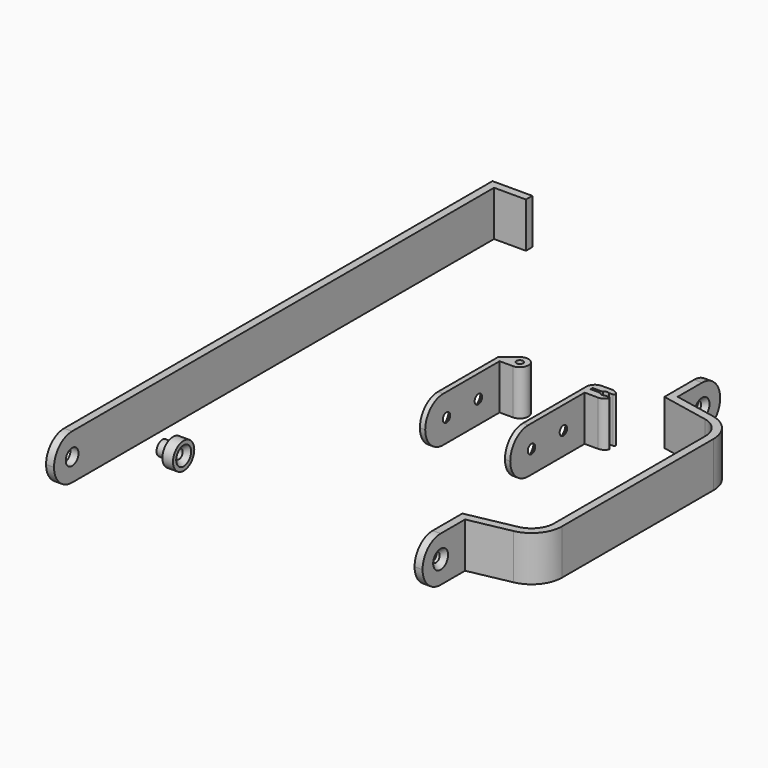
from build123d import *

# Parameters (mm, degrees)
F0_R                 = 1.25
F1_DEPTH             = 17
F4_R                 = 8.49999
F4_2_R               = 8.49999
F4_3_R               = 8.49999
F4_4_R               = 8.49999
F5_R                 = 0.5
F7_D                 = 3.5
F7_DEPTH             = 20
F7_CSINK_D           = 7
F7_CSINK_ANGLE       = 90
F7_TIP               = 1.0515060833
F7_ON_F3_D           = 3.5
F7_ON_F3_DEPTH       = 20
F7_ON_F3_CSINK_D     = 7
F7_ON_F3_CSINK_ANGLE = 90
F7_ON_F3_TIP         = 1.0515060833
F7_ON_F6_D           = 3.5
F7_ON_F6_DEPTH       = 20
F7_ON_F6_CSINK_D     = 7
F7_ON_F6_CSINK_ANGLE = 90
F7_ON_F6_TIP         = 1.0515060833
F8_R                 = 11.5
F9_R                 = 3
F10_DEPTH            = 25
F14_D                = 3.5
F14_DEPTH            = 20
F14_CSINK_D          = 7
F14_CSINK_ANGLE      = 90
F14_TIP              = 1.0515060833


# Not quite as in the source:
# - a fillet or chamfer is up to 0.001 mm smaller than in the source, because OpenCascade refuses the exact size


with BuildPart() as f1:
    # F0 (on Top) → F1 (new body)
    with BuildSketch(Plane.XY):
        with BuildLine():
            Line((1, 17.5), (6, 17.5))
            ThreePointArc((6, 17.5), (9.0791424151, 21.7898951811), (4.0295474712, 23.3345341614))
            Line((4.0295474712, 23.3345341614), (-1, 19.5))
            Line((-1, 19.5), (-1, -17.5))
            Line((-1, -17.5), (1, -17.5))
            Line((1, -17.5), (1, 17.5))
        make_face()
        with Locations((6, 20.75)):
            Circle(F0_R, mode=Mode.SUBTRACT)
    extrude(amount=F1_DEPTH)

    # F4 (radius 8.5 in the source; OpenCascade refuses exactly that, so slightly less here)
    f4_edges = [f1.edges().sort_by_distance(p)[0] for p in [
        (0, -17.5, 17),
        (0, -17.5, 0),
    ]]
    fillet(f4_edges, radius=F4_R)

    # F7
    with Locations(Plane(origin=(-1, 0, 0), x_dir=(0, -1, 0), z_dir=(-1, 0, 0))):
        with Locations((7.5, 8.5), (-7.5, 8.5)):
            CounterSinkHole(F7_D / 2, F7_CSINK_D / 2, depth=F7_DEPTH, counter_sink_angle=F7_CSINK_ANGLE)
            with Locations((0, 0, -(F7_DEPTH + F7_TIP / 2))):  # 118° drill point
                Cone(0, F7_D / 2, F7_TIP, mode=Mode.SUBTRACT)


with BuildPart() as f1b:
    # F0 (on Top) → F1, piece 2 (new body)
    with BuildSketch(Plane.XY):
        with BuildLine():
            Line((33, 17.5), (38, 17.5))
            ThreePointArc((38, 17.5), (39.9121323176, 18.1220254948), (41.0923292192, 19.75))
            Line((41.0923292192, 19.75), (38.75, 19.75))
            ThreePointArc((38.75, 19.75), (37.681199861, 19.5413369074), (36.8543560763, 20.25))
            Line((36.8543560763, 20.25), (33, 20.25))
            Line((33, 20.25), (33, 21.25))
            Line((33, 21.25), (36.8543560763, 21.25))
            ThreePointArc((36.8543560763, 21.25), (37.681199861, 21.9586630926), (38.75, 21.75))
            Line((38.75, 21.75), (41.0923292192, 21.75))
            ThreePointArc((41.0923292192, 21.75), (39.9121323176, 23.3779745052), (38, 24))
            Line((38, 24), (34.25, 24))
            ThreePointArc((34.25, 24), (31.9519029611, 23.0480970389), (31, 20.75))
            Line((31, 20.75), (31, -17.5))
            Line((31, -17.5), (33, -17.5))
            Line((33, -17.5), (33, 17.5))
        make_face()
    extrude(amount=F1_DEPTH)

    # F4#2 (radius 8.5 in the source; OpenCascade refuses exactly that, so slightly less here)
    f4_2_edges = [f1b.edges().sort_by_distance(p)[0] for p in [
        (32, -17.5, 17),
        (32, -17.5, 0),
    ]]
    fillet(f4_2_edges, radius=F4_2_R)

    # F5
    f5_edges = [f1b.edges().sort_by_distance(p)[0] for p in [
        (41.092329, 19.75, 8.5),
        (41.092329, 21.75, 8.5),
    ]]
    fillet(f5_edges, radius=F5_R)

    # F7 on F3
    with Locations(Plane(origin=(31, 0, 0), x_dir=(0, -1, 0), z_dir=(-1, 0, 0))):
        with Locations((7.5, 8.5), (-7.5, 8.5)):
            CounterSinkHole(F7_ON_F3_D / 2, F7_ON_F3_CSINK_D / 2, depth=F7_ON_F3_DEPTH, counter_sink_angle=F7_ON_F3_CSINK_ANGLE)
            with Locations((0, 0, -(F7_ON_F3_DEPTH + F7_ON_F3_TIP / 2))):  # 118° drill point
                Cone(0, F7_ON_F3_D / 2, F7_ON_F3_TIP, mode=Mode.SUBTRACT)


with BuildPart() as f1c:
    # F0 (on Top) → F1, piece 3 (new body)
    with BuildSketch(Plane.XY):
        Polygon((56, 32.5), (56, 52.5), (53, 52.5), (53, 30.0405882918), (78, 25.0405882918), (78, -17.5), (78, -60.0405882918), (53, -65.0405882918), (53, -87.5), (56, -87.5), (56, -67.5), (81, -62.5), (81, -17.5), (81, 27.5), align=None)
    extrude(amount=F1_DEPTH)

    # F4#3 (radius 8.5 in the source; OpenCascade refuses exactly that, so slightly less here)
    f4_3_edges = [f1c.edges().sort_by_distance(p)[0] for p in [
        (54.5, 52.5, 17),
        (54.5, 52.5, 0),
        (54.5, -87.5, 17),
        (54.5, -87.5, 0),
        (78, -60.040588, 8.5),
        (78, 25.040588, 8.5),
    ]]
    fillet(f4_3_edges, radius=F4_3_R)

    # F7 on F6
    with Locations(Plane.YZ.offset(56)):
        with Locations((44, 8.5), (-79, 8.5)):
            CounterSinkHole(F7_ON_F6_D / 2, F7_ON_F6_CSINK_D / 2, depth=F7_ON_F6_DEPTH, counter_sink_angle=F7_ON_F6_CSINK_ANGLE)
            with Locations((0, 0, -(F7_ON_F6_DEPTH + F7_ON_F6_TIP / 2))):  # 118° drill point
                Cone(0, F7_ON_F6_D / 2, F7_ON_F6_TIP, mode=Mode.SUBTRACT)

    # F8
    f8_edges = [f1c.edges().sort_by_distance(p)[0] for p in [
        (81, -62.5, 8.5),
        (81, 27.5, 8.5),
    ]]
    fillet(f8_edges, radius=F8_R)


with BuildPart() as f1d:
    # F0 (on Top) → F1, piece 4 (new body)
    with BuildSketch(Plane.XY):
        Polygon((-72.2447633743, 105.6920430064), (-72.2447633743, -104.3079569936), (-69.2447633743, -104.3079569936), (-69.2447633743, 102.6920430064), (-57.2447633743, 102.6920430064), (-57.2447633743, 105.6920430064), align=None)
    extrude(amount=F1_DEPTH)

    # F4#4 (radius 8.5 in the source; OpenCascade refuses exactly that, so slightly less here)
    f4_4_edges = [f1d.edges().sort_by_distance(p)[0] for p in [
        (-70.744763, -104.307957, 17),
        (-70.744763, -104.307957, 0),
    ]]
    fillet(f4_4_edges, radius=F4_4_R)

    # F9 (on face) → F10 (cut)
    with BuildSketch(Plane.YZ.offset(-69.2447633743)):
        with Locations((-95.8079569936, 8.5)):
            Circle(F9_R)
    extrude(amount=-F10_DEPTH, mode=Mode.SUBTRACT)


with BuildPart() as f12:
    # F11 (on Top) → F12 (revolve)
    with BuildSketch(Plane.XY):
        Polygon((-62.2995859704, -59.2756714114), (-62.2995859704, -62.0256714114), (-54.2995859704, -62.0256714114), (-54.2995859704, -57.0256714114), (-58.2995859704, -57.0256714114), (-58.2995859704, -59.2756714114), align=None)
    revolve(axis=Axis((-56.4878471196, -62.0256714114, 0), (1, 0, 0)))

    # F14
    with Locations(Plane.YZ.offset(-54.2995859704)):
        with Locations((-62.0256714114, 0)):
            CounterSinkHole(F14_D / 2, F14_CSINK_D / 2, depth=F14_DEPTH, counter_sink_angle=F14_CSINK_ANGLE)
            with Locations((0, 0, -(F14_DEPTH + F14_TIP / 2))):  # 118° drill point
                Cone(0, F14_D / 2, F14_TIP, mode=Mode.SUBTRACT)


solid = Compound([f1.part, f1b.part, f1c.part, f1d.part, f12.part])
